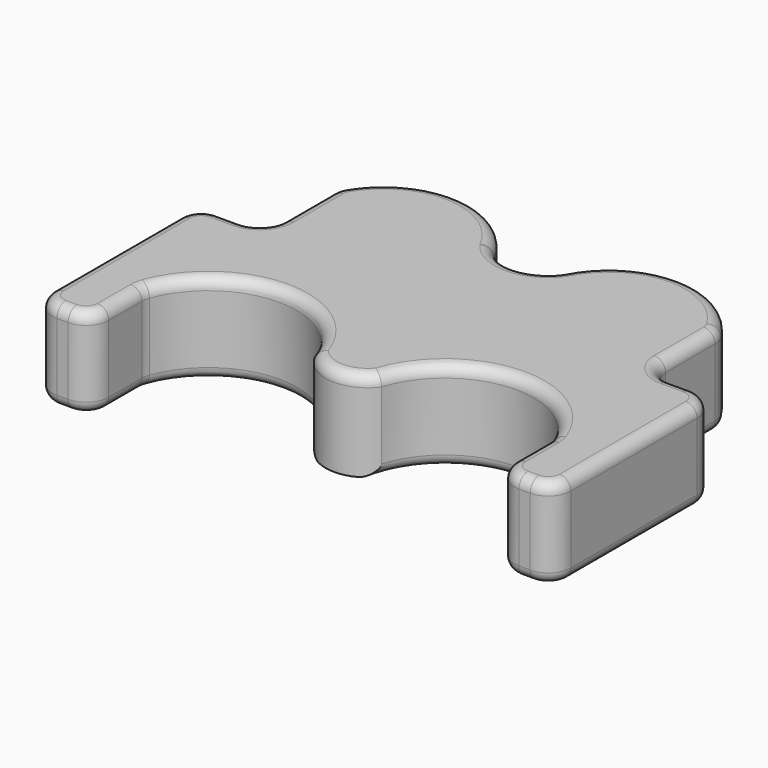
from build123d import *

# Parameters (mm, degrees)
F1_DEPTH = 4
F2_R     = 1
F3_R     = 0.5


# Not quite as in the source:
# - a feature names something its author has since deleted; it is built from what else it names


with BuildPart() as f1:
    # F0 (on Top) → F1 (new body)
    with BuildSketch(Plane.XY):
        with BuildLine():
            Line((9, -10), (9, -13))
            Line((9, -13), (11.5, -13))
            Line((11.5, -13), (11.5, -4))
            Line((11.5, -4), (8.5, -4))
            Line((8.5, -4), (8.5, 0))
            ThreePointArc((8.5, 0), (5, 2.1457607663), (1.5, 0))
            ThreePointArc((1.5, 0), (0, -0.7515530935), (-1.5, 0))
            ThreePointArc((-1.5, 0), (-5, 2.1457607663), (-8.5, 0))
            Line((-8.5, 0), (-8.5, -4))
            Line((-8.5, -4), (-11.5, -4))
            Line((-11.5, -4), (-11.5, -13))
            Line((-11.5, -13), (-9, -13))
            Line((-9, -13), (-9, -10))
            ThreePointArc((-9, -10), (-5.25, -7.2395069282), (-1.5, -10))
            ThreePointArc((-1.5, -10), (0, -10.7515530935), (1.5, -10))
            ThreePointArc((1.5, -10), (5.25, -7.2395069282), (9, -10))
        make_face()
    extrude(amount=F1_DEPTH)

    # F2
    f2_edges = [f1.edges().sort_by_distance(p)[0] for p in [
        (-9, -13, 2),
        (9, -13, 2),
        (-11.5, -4, 2),
        (-8.5, -4, 2),
        (8.5, -4, 2),
        (11.5, -4, 2),
        (9, -10, 2),
        (11.5, -13, 2),
        (8.5, 0, 2),
        (-8.5, 0, 2),
        (-11.5, -13, 2),
        (-9, -10, 2),
    ]]
    fillet(f2_edges, radius=F2_R)

    # F3 (call 1 of 2: OpenCascade refuses the feature's edges together)
    f3_edges = [f1.edges().sort_by_distance(p)[0] for p in [
        (-4.85021, 2.142903, 4),
        (-8.462813, 0.011528, 4),
        (-8.5, -1.629321, 4),
        (-8.792893, -3.707107, 4),
        (-10, -4, 4),
        (-11.207107, -4.292893, 4),
        (-11.5, -8.5, 4),
        (-11.207107, -12.707107, 4),
        (-10.25, -13, 4),
        (-9.292893, -12.707107, 4),
        (-9, -11.081716, 4),
        (-5.15535, -7.240648, 4),
        (-8.984738, -9.989388, 4),
        (0, -10.751553, 4),
        (5.15535, -7.240648, 4),
        (8.984738, -9.989388, 4),
        (9, -11.081716, 4),
        (9.292893, -12.707107, 4),
        (10.25, -13, 4),
        (11.207107, -12.707107, 4),
        (11.5, -8.5, 4),
        (10, -4, 4),
        (8.792893, -3.707107, 4),
        (11.207107, -4.292893, 4),
        (8.5, -1.629321, 4),
        (8.462813, 0.011528, 4),
        (4.85021, 2.142903, 4),
        (0, -0.751553, 4),
    ]]
    fillet(f3_edges, radius=F3_R)

    # F3#2 (call 2 of 2)
    f3_2_edges = [f1.edges().sort_by_distance(p)[0] for p in [
        (4.85021, 2.142903, 0),
        (0, -0.751553, 0),
        (-4.85021, 2.142903, 0),
        (-8.462813, 0.011528, 0),
        (-8.5, -1.629321, 0),
        (-8.792893, -3.707107, 0),
        (-10, -4, 0),
        (5.15535, -7.240648, 0),
        (8.984738, -9.989388, 0),
        (9, -11.081716, 0),
        (-5.15535, -7.240648, 0),
        (9.292893, -12.707107, 0),
        (-8.984738, -9.989388, 0),
        (10.25, -13, 0),
        (-9, -11.081716, 0),
        (11.207107, -12.707107, 0),
        (-9.292893, -12.707107, 0),
        (11.5, -8.5, 0),
        (-10.25, -13, 0),
        (11.207107, -4.292893, 0),
        (-11.207107, -12.707107, 0),
        (10, -4, 0),
        (-11.5, -8.5, 0),
        (8.792893, -3.707107, 0),
        (-11.207107, -4.292893, 0),
        (8.5, -1.629321, 0),
        (8.462813, 0.011528, 0),
    ]]
    fillet(f3_2_edges, radius=F3_R)


solid = f1.part
